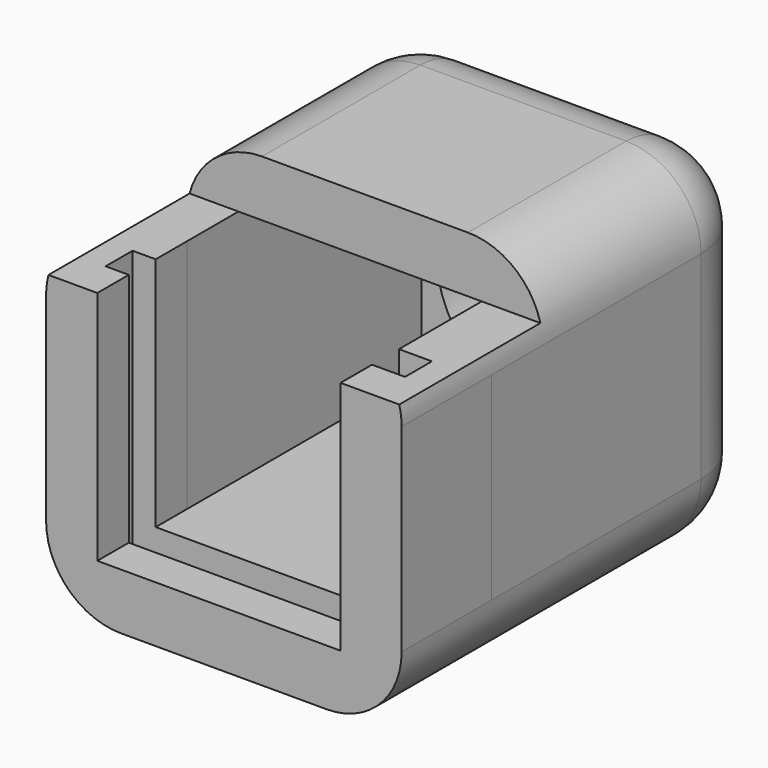
from build123d import *

# Parameters (mm, degrees)
F0_W         = 1.3692331631
F0_H         = 7.834737435
F0_W_2       = 6.5
F0_H_2       = 0.9
F0_W_3       = 0.6192331631
F0_H_3       = 1.05
F0_H_4       = 1.165262565
F0_W_4       = 0.8807668369
F0_W_5       = 1.6307668369
F1_DEPTH     = 0.9
F2_DEPTH     = 1.5
F3_DEPTH     = 7.8
F5_W         = 9.5
F5_H         = 7.2867757659
F6_DEPTH     = 1.5
F7_R         = 3
F8_DEPTH     = 10.501
F9_T1_DEPTH  = 5.3
F9_T3_DEPTH  = 5.5
F9_T5_DEPTH  = 10.2867757659
F9_T7_DEPTH  = 15
F9_S11_W     = 2
F9_S11_H     = 2
F9_T12_DEPTH = 2
F9_S17_W     = 2
F9_S17_H     = 2
F9_T18_DEPTH = 2
F9_S23_W     = 2
F9_S23_H     = 2
F9_T24_DEPTH = 2
F9_S29_W     = 2
F9_S29_H     = 2
F9_T30_DEPTH = 2


# Not quite as in the source:
# - a fillet or chamfer that OpenCascade refuses, or shapes differently, is made with other operations: its cross-section is extruded or revolved along the edge and cut away or added
# - a feature names something its author has since deleted; it is built from what else it names


with BuildPart() as f1:
    # F0 (on Top) → F1 (new body)
    with BuildSketch(Plane.XY):
        Polygon((-4.75, 1.5), (-4.75, -1.5), (-3.3807668369, -1.5), (-3.3807668369, -0.45), (-4, -0.45), (-4, 0.45), (-3.3807668369, 0.45), (-3.3807668369, 1.5), align=None)
        Polygon((-3.3807668369, -0.45), (-3.3807668369, -1.5), (-3.1192331631, -1.5), (3.1192331631, -1.5), (3.1192331631, -0.45), align=None)
        with Locations((-4.0653834185, 5.4173687175)):
            Rectangle(F0_W, F0_H)
        with Locations((-0.1307668369, 0)):
            Rectangle(F0_W_2, F0_H_2)
        with Locations((-3.6903834185, 0)):
            Rectangle(F0_W_3, F0_H_2)
        with Locations((-0.1307668369, 5.4173687175)):
            Rectangle(F0_W_2, F0_H)
        with Locations((-0.1307668369, 0.975)):
            Rectangle(F0_W_2, F0_H_3)
        with Locations((-4.0653834185, 9.9173687175)):
            Rectangle(F0_W, F0_H_4)
        Polygon((3.1192331631, -0.45), (3.1192331631, -1.5), (3.3807668369, -1.5), (4.75, -1.5), (4.75, 1.5), (3.1192331631, 1.5), (3.1192331631, 0.45), (4, 0.45), (4, -0.45), align=None)
        with Locations((3.5596165815, 0)):
            Rectangle(F0_W_4, F0_H_2)
        with Locations((3.9346165815, 5.4173687175)):
            Rectangle(F0_W_5, F0_H)
        with Locations((-0.1307668369, 9.9173687175)):
            Rectangle(F0_W_2, F0_H_4)
        with Locations((3.9346165815, 9.9173687175)):
            Rectangle(F0_W_5, F0_H_4)
    extrude(amount=F1_DEPTH)

    # F0 (on Top) → F2 (join)
    with BuildSketch(Plane.XY):
        Polygon((-3.3807668369, -0.45), (-3.3807668369, -1.5), (-3.1192331631, -1.5), (3.1192331631, -1.5), (3.1192331631, -0.45), align=None)
        Polygon((3.1192331631, -0.45), (3.1192331631, -1.5), (3.3807668369, -1.5), (4.75, -1.5), (4.75, 1.5), (3.1192331631, 1.5), (3.1192331631, 0.45), (4, 0.45), (4, -0.45), align=None)
        Polygon((-4.75, 1.5), (-4.75, -1.5), (-3.3807668369, -1.5), (-3.3807668369, -0.45), (-4, -0.45), (-4, 0.45), (-3.3807668369, 0.45), (-3.3807668369, 1.5), align=None)
        with Locations((-0.1307668369, 0.975)):
            Rectangle(F0_W_2, F0_H_3)
        with Locations((-4.0653834185, 5.4173687175)):
            Rectangle(F0_W, F0_H)
        with Locations((3.9346165815, 5.4173687175)):
            Rectangle(F0_W_5, F0_H)
        with Locations((-0.1307668369, 5.4173687175)):
            Rectangle(F0_W_2, F0_H)
        with Locations((-4.0653834185, 9.9173687175)):
            Rectangle(F0_W, F0_H_4)
        with Locations((-0.1307668369, 9.9173687175)):
            Rectangle(F0_W_2, F0_H_4)
        with Locations((3.9346165815, 9.9173687175)):
            Rectangle(F0_W_5, F0_H_4)
    extrude(amount=F2_DEPTH)

    # F0 (on Top) → F3 (join)
    with BuildSketch(Plane.XY):
        Polygon((-4.75, 1.5), (-4.75, -1.5), (-3.3807668369, -1.5), (-3.3807668369, -0.45), (-4, -0.45), (-4, 0.45), (-3.3807668369, 0.45), (-3.3807668369, 1.5), align=None)
        Polygon((3.1192331631, -0.45), (3.1192331631, -1.5), (3.3807668369, -1.5), (4.75, -1.5), (4.75, 1.5), (3.1192331631, 1.5), (3.1192331631, 0.45), (4, 0.45), (4, -0.45), align=None)
        with Locations((-4.0653834185, 5.4173687175)):
            Rectangle(F0_W, F0_H)
        with Locations((3.9346165815, 5.4173687175)):
            Rectangle(F0_W_5, F0_H)
        with Locations((-4.0653834185, 9.9173687175)):
            Rectangle(F0_W, F0_H_4)
        with Locations((-0.1307668369, 9.9173687175)):
            Rectangle(F0_W_2, F0_H_4)
        with Locations((3.9346165815, 9.9173687175)):
            Rectangle(F0_W_5, F0_H_4)
    extrude(amount=F3_DEPTH)

    # F5 (on offset) → F6 (join)
    with BuildSketch(Plane.XY.offset(7.8)):
        with Locations((0, 6.856612117)):
            Rectangle(F5_W, F5_H)
    extrude(amount=F6_DEPTH)

    # F7 (on Front) → F8 (cut, through all)
    with BuildSketch(Plane.XZ):
        with Locations((0, 4.5)):
            Circle(F7_R)
    extrude(amount=-F8_DEPTH, mode=Mode.SUBTRACT)

    # F9: fillet of radius 2 on 8 edges, made by hand

    # F9_s2 → F9_t1 (cut)
    with BuildSketch(Plane.XY.offset(2)):
        with BuildLine():
            ThreePointArc((4.75, 8.5), (4.1642135624, 9.9142135624), (2.75, 10.5))
            Line((2.75, 10.5), (4.75, 10.5))
            Line((4.75, 10.5), (4.75, 8.5))
        make_face()
        with BuildLine():
            ThreePointArc((-4.75, 8.5), (-4.1642135624, 9.9142135624), (-2.75, 10.5))
            Line((-2.75, 10.5), (-4.75, 10.5))
            Line((-4.75, 10.5), (-4.75, 8.5))
        make_face()
    extrude(amount=F9_T1_DEPTH, mode=Mode.SUBTRACT)

    # F9_s4 → F9_t3 (cut)
    with BuildSketch(Plane.YZ.offset(-2.75)):
        with BuildLine():
            ThreePointArc((8.5, 9.3), (9.9142135624, 8.7142135624), (10.5, 7.3))
            Line((10.5, 7.3), (10.5, 9.3))
            Line((10.5, 9.3), (8.5, 9.3))
        make_face()
        with BuildLine():
            ThreePointArc((8.5, 0), (9.9142135624, 0.5857864376), (10.5, 2))
            Line((10.5, 2), (10.5, 0))
            Line((10.5, 0), (8.5, 0))
        make_face()
    extrude(amount=F9_T3_DEPTH, mode=Mode.SUBTRACT)

    # F9_s6 → F9_t5 (cut)
    with BuildSketch(Plane.XZ.offset(-8.5)):
        with BuildLine():
            ThreePointArc((4.75, 7.3), (4.1642135624, 8.7142135624), (2.75, 9.3))
            Line((2.75, 9.3), (4.75, 9.3))
            Line((4.75, 9.3), (4.75, 7.3))
        make_face()
        with BuildLine():
            ThreePointArc((-4.75, 7.3), (-4.1642135624, 8.7142135624), (-2.75, 9.3))
            Line((-2.75, 9.3), (-4.75, 9.3))
            Line((-4.75, 9.3), (-4.75, 7.3))
        make_face()
    extrude(amount=F9_T5_DEPTH, mode=Mode.SUBTRACT)

    # F9_s8 → F9_t7 (cut)
    with BuildSketch(Plane.XZ.offset(-8.5)):
        with BuildLine():
            ThreePointArc((2.75, 0), (4.1642135624, 0.5857864376), (4.75, 2))
            Line((4.75, 2), (4.75, 0))
            Line((4.75, 0), (2.75, 0))
        make_face()
        with BuildLine():
            ThreePointArc((-4.75, 2), (-4.1642135624, 0.5857864376), (-2.75, 0))
            Line((-2.75, 0), (-4.75, 0))
            Line((-4.75, 0), (-4.75, 2))
        make_face()
    extrude(amount=F9_T7_DEPTH, mode=Mode.SUBTRACT)


with BuildPart() as f9_tool10:
    # F9_s11 → F9_t12 (new body)
    with BuildSketch(Plane.YZ.offset(2.75)):
        with Locations((9.5, 8.3)):
            Rectangle(F9_S11_W, F9_S11_H)
    extrude(amount=F9_T12_DEPTH)

    # F9_s13 → F9_t14 (revolve, cut)
    with BuildSketch(Plane(origin=(2.75, 8.5, 7.3), x_dir=(0, -0.7071067812, -0.7071067812), z_dir=(0, -0.7071067812, 0.7071067812))):
        with BuildLine():
            ThreePointArc((0, -2), (2, 0), (0, 2))
            Line((0, 2), (0, -2))
        make_face()
    revolve(axis=Axis((2.75, 8.5, 7.3), (1, 0, 0)), mode=Mode.SUBTRACT)


with BuildPart() as f1_1:
    add(f1.part)

    # F9_t9: cut F9_tool10
    add(f9_tool10.part, mode=Mode.SUBTRACT)


with BuildPart() as f9_tool16:
    # F9_s17 → F9_t18 (new body)
    with BuildSketch(Plane.XY.offset(2)):
        with Locations((3.75, 9.5)):
            Rectangle(F9_S17_W, F9_S17_H)
    extrude(amount=-F9_T18_DEPTH)

    # F9_s19 → F9_t20 (revolve, cut)
    with BuildSketch(Plane(origin=(2.75, 8.5, 2), x_dir=(-0.7071067812, -0.7071067812, 0), z_dir=(0.7071067812, -0.7071067812, 0))):
        with BuildLine():
            ThreePointArc((0, -2), (2, 0), (0, 2))
            Line((0, 2), (0, -2))
        make_face()
    revolve(axis=Axis((2.75, 8.5, 2), (0, 0, -1)), mode=Mode.SUBTRACT)


with BuildPart() as f1_2:
    add(f1_1.part)

    # F9_t15: cut F9_tool16
    add(f9_tool16.part, mode=Mode.SUBTRACT)


with BuildPart() as f9_tool22:
    # F9_s23 → F9_t24 (new body)
    with BuildSketch(Plane.YZ.offset(-2.75)):
        with Locations((9.5, 8.3)):
            Rectangle(F9_S23_W, F9_S23_H)
    extrude(amount=-F9_T24_DEPTH)

    # F9_s25 → F9_t26 (revolve, cut)
    with BuildSketch(Plane(origin=(-2.75, 8.5, 7.3), x_dir=(0, -0.7071067812, -0.7071067812), z_dir=(0, 0.7071067812, -0.7071067812))):
        with BuildLine():
            ThreePointArc((0, -2), (2, 0), (0, 2))
            Line((0, 2), (0, -2))
        make_face()
    revolve(axis=Axis((-2.75, 8.5, 7.3), (-1, 0, 0)), mode=Mode.SUBTRACT)


with BuildPart() as f1_3:
    add(f1_2.part)

    # F9_t21: cut F9_tool22
    add(f9_tool22.part, mode=Mode.SUBTRACT)


with BuildPart() as f9_tool28:
    # F9_s29 → F9_t30 (new body)
    with BuildSketch(Plane.YZ.offset(-2.75)):
        with Locations((9.5, 1)):
            Rectangle(F9_S29_W, F9_S29_H)
    extrude(amount=-F9_T30_DEPTH)

    # F9_s31 → F9_t32 (revolve, cut)
    with BuildSketch(Plane(origin=(-2.75, 8.5, 2), x_dir=(0, -0.7071067812, 0.7071067812), z_dir=(0, -0.7071067812, -0.7071067812))):
        with BuildLine():
            ThreePointArc((0, -2), (2, 0), (0, 2))
            Line((0, 2), (0, -2))
        make_face()
    revolve(axis=Axis((-2.75, 8.5, 2), (-1, 0, 0)), mode=Mode.SUBTRACT)


with BuildPart() as f1_4:
    add(f1_3.part)

    # F9_t27: cut F9_tool28
    add(f9_tool28.part, mode=Mode.SUBTRACT)


solid = f1_4.part
